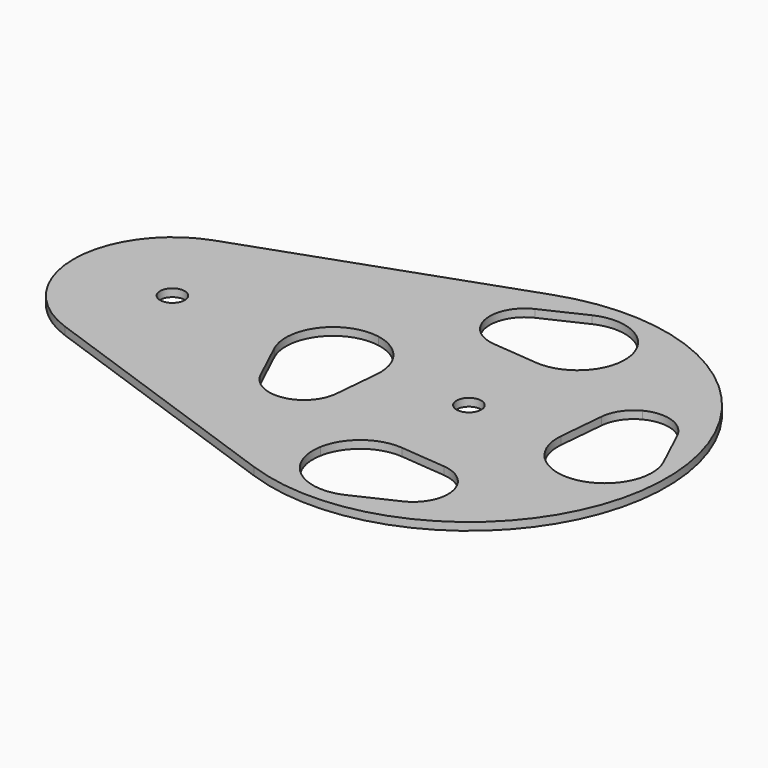
from build123d import *

# Parameters (mm, degrees)
F0_R            = 3.175
F1_DEPTH        = 2
F3_DEPTH        = 2.001
F3_COPIES_COUNT = 4


# Not quite as in the source:
# - a pattern or mirror of a feature is missing from the dataset's text; its kind, count and spacing are read off the source's solid


with BuildPart() as f1:
    # F0 (on Top) → F1 (new body)
    with BuildSketch(Plane.XY):
        with BuildLine():
            Line((-84.6666666667, -23.9473496562), (-16.9333333333, -47.8946993124))
            ThreePointArc((-16.9333333333, -47.8946993124), (50.8, 0), (-16.9333333333, 47.8946993124))
            Line((-16.9333333333, 47.8946993124), (-84.6666666667, 23.9473496562))
            ThreePointArc((-84.6666666667, 23.9473496562), (-101.6, 0), (-84.6666666667, -23.9473496562))
        make_face()
        with Locations((-76.2, 0)):
            Circle(F0_R, mode=Mode.SUBTRACT)
        Circle(F0_R, mode=Mode.SUBTRACT)
    extrude(amount=F1_DEPTH)

    # F2 (on face) → F3 (cut, through all)
    with BuildSketch(Plane.XY.offset(2)):
        with BuildLine():
            ThreePointArc((-28.7020344674, -19.8984633183), (-34.6367957344, -4.4775), (-32.8185304223, 11.945697381))
            ThreePointArc((-32.8185304223, 11.945697381), (-44.5595640794, 7.3696726522), (-45.9028628242, -5.1597895126))
            Line((-45.9028628242, -5.1597895126), (-40.9229625402, -15.7549236864))
            ThreePointArc((-40.9229625402, -15.7549236864), (-35.6939675857, -20.4264925159), (-28.7020344674, -19.8984633183))
        make_face()
        with BuildLine():
            ThreePointArc((-22.8444099031, -1.093728902), (-25.2904359206, 7.3696726522), (-32.8185304223, 11.945697381))
            ThreePointArc((-32.8185304223, 11.945697381), (-34.6367957344, -4.4775), (-28.7020344674, -19.8984633183))
            ThreePointArc((-28.7020344674, -19.8984633183), (-25.386046138, -16.940715135), (-23.9000073953, -12.7531452225))
            Line((-23.9000073953, -12.7531452225), (-22.8444099031, -1.093728902))
        make_face()
    f3 = extrude(amount=-F3_DEPTH, mode=Mode.SUBTRACT)

    # F3_copies: F3 ×4 about axis
    f3_copies_axis = Axis((0, 0, 0), (0, 0, 1))
    for i in range(1, F3_COPIES_COUNT):
        add(f3.rotate(f3_copies_axis, i * 360 / F3_COPIES_COUNT), mode=Mode.SUBTRACT)


solid = f1.part
